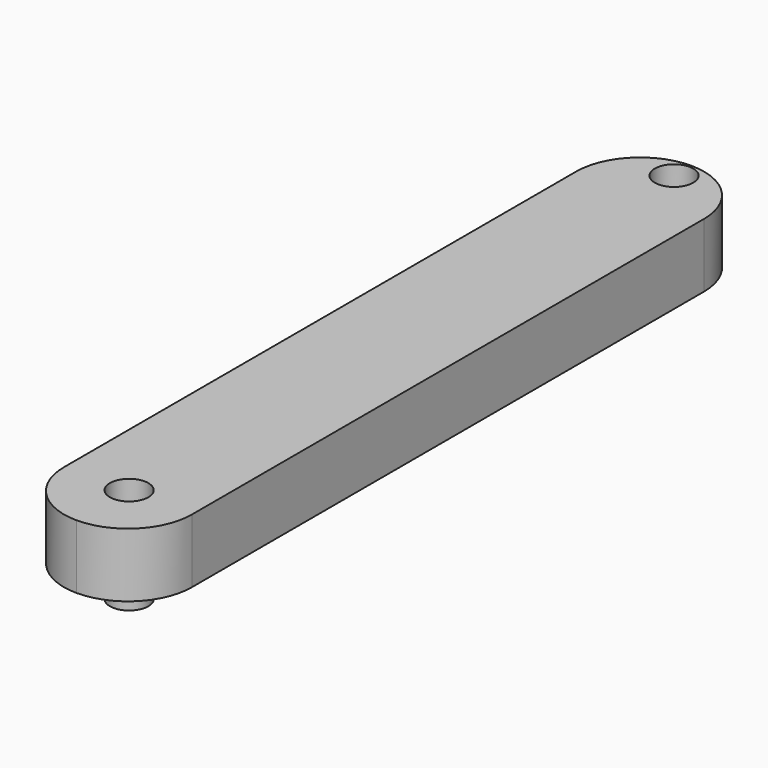
from build123d import *

# Parameters (mm, degrees)
F0_W     = 10
F0_H     = 60
F0_R     = 1.5
F1_DEPTH = 2.5
F2_DEPTH = 5
F3_R     = 4.99999


# Not quite as in the source:
# - a fillet or chamfer is up to 0.001 mm smaller than in the source, because OpenCascade refuses the exact size


with BuildPart() as f1:
    # F0 (on Top) → F1 (new body, symmetric)
    with BuildSketch(Plane.XY):
        with Locations((-32.8091010451, 20.9925968945)):
            Rectangle(F0_W, F0_H)
        with Locations((-32.8091010451, -3.8919287648)):
            Circle(F0_R, mode=Mode.SUBTRACT)
        with Locations((-32.8091010451, 49.3113994598)):
            Circle(F0_R, mode=Mode.SUBTRACT)
    extrude(amount=F1_DEPTH, both=True)

    # F0 (on Top) → F2 (join)
    with BuildSketch(Plane.XY):
        with Locations((-32.8091010451, 49.3113994598)):
            Circle(F0_R)
        with Locations((-32.8091010451, -3.8919287648)):
            Circle(F0_R)
    extrude(amount=-F2_DEPTH)

    # F3 (radius 5 in the source; OpenCascade refuses exactly that, so slightly less here)
    f3_edges = [f1.edges().sort_by_distance(p)[0] for p in [
        (-27.809101, 50.992597, 0),
        (-37.809101, 50.992597, 0),
        (-27.809101, -9.007403, 0),
        (-37.809101, -9.007403, 0),
    ]]
    fillet(f3_edges, radius=F3_R)


solid = f1.part
